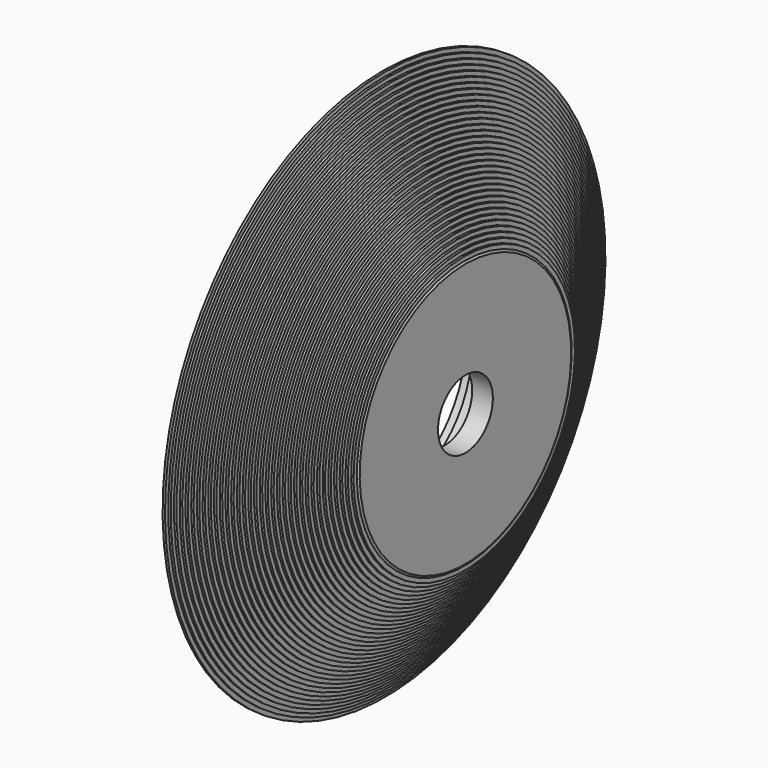
from build123d import *

# Parameters (mm, degrees)
F1_W     = 2.5
F1_H     = 6.85
F3_R     = 12.7
F3_R_2   = 11
F4_DEPTH = 2


# Not quite as in the source:
# - a feature names something its author has since deleted; it is built from what else it names


with BuildPart() as f2:
    # F1 (on Front) → F2 (revolve)
    with BuildSketch(Plane.XZ):
        Polygon((0, 33.3265457083), (0, 11), (7.5, 11), (10, 11), (10, 16), (9.8575705779, 16.2527326282), (9.8575705779, 16.7527326282), (9.5676420315, 16.7549036012), (9.5676420315, 17.2549036012), (9.2777134851, 17.2570745741), (9.2777134851, 17.7570745741), (8.9877849387, 17.759245547), (8.9877849387, 18.259245547), (8.6978563922, 18.26141652), (8.6978563922, 18.76141652), (8.4079278458, 18.7635874929), (8.4079278458, 19.2635874929), (8.1179992994, 19.2657584659), (8.1179992994, 19.7657584659), (7.828070753, 19.7679294388), (7.828070753, 20.2679294388), (7.5381422066, 20.2701004118), (7.5381422066, 20.7701004118), (7.2482136602, 20.7722713847), (7.2482136602, 21.2722713847), (6.9582851138, 21.2744423577), (6.9582851138, 21.7744423577), (6.6683565674, 21.7766133306), (6.6683565674, 22.2766133306), (6.378428021, 22.2787843035), (6.378428021, 22.7787843035), (6.0884994746, 22.7809552765), (6.0884994746, 23.2809552765), (5.7985709282, 23.2831262494), (5.7985709282, 23.7831262494), (5.5086423818, 23.7852972224), (5.5086423818, 24.2852972224), (5.2187138353, 24.2874681953), (5.2187138353, 24.7874681953), (4.9287852889, 24.7896391683), (4.9287852889, 25.2896391683), (4.6388567425, 25.2918101412), (4.6388567425, 25.7918101412), (4.3489281961, 25.7939811141), (4.3489281961, 26.2939811141), (4.0589996497, 26.2961520871), (4.0589996497, 26.7961520871), (3.7690711033, 26.79832306), (3.7690711033, 27.29832306), (3.4791425569, 27.300494033), (3.4791425569, 27.800494033), (3.1892140105, 27.8026650059), (3.1892140105, 28.3026650059), (2.8992854641, 28.3048359789), (2.8992854641, 28.8048359789), (2.6093569177, 28.8070069518), (2.6093569177, 29.3070069518), (2.3194283713, 29.3091779248), (2.3194283713, 29.8091779248), (2.0294998249, 29.8113488977), (2.0294998249, 30.3113488977), (1.7395712784, 30.3135198706), (1.7395712784, 30.8135198706), (1.449642732, 30.8156908436), (1.449642732, 31.3156908436), (1.1597141856, 31.3178618165), (1.1597141856, 31.8178618165), (0.8697856392, 31.8200327895), (0.8697856392, 32.3200327895), (0.5798570928, 32.3222037624), (0.5798570928, 32.8222037624), (0.2899285464, 32.8243747354), (0.2899285464, 33.3243747354), align=None)
        with Locations((8.75, 7.575)):
            Rectangle(F1_W, F1_H)
    revolve(axis=Axis((0, 0, 0), (1, 0, 0)))

    # F3 (on face) → F4 (cut)
    with BuildSketch(Plane(origin=(0, 0, 0), x_dir=(0, -1, 0), z_dir=(-1, 0, 0))):
        Circle(F3_R)
        Circle(F3_R_2, mode=Mode.SUBTRACT)
    extrude(amount=-F4_DEPTH, mode=Mode.SUBTRACT)


solid = f2.part
